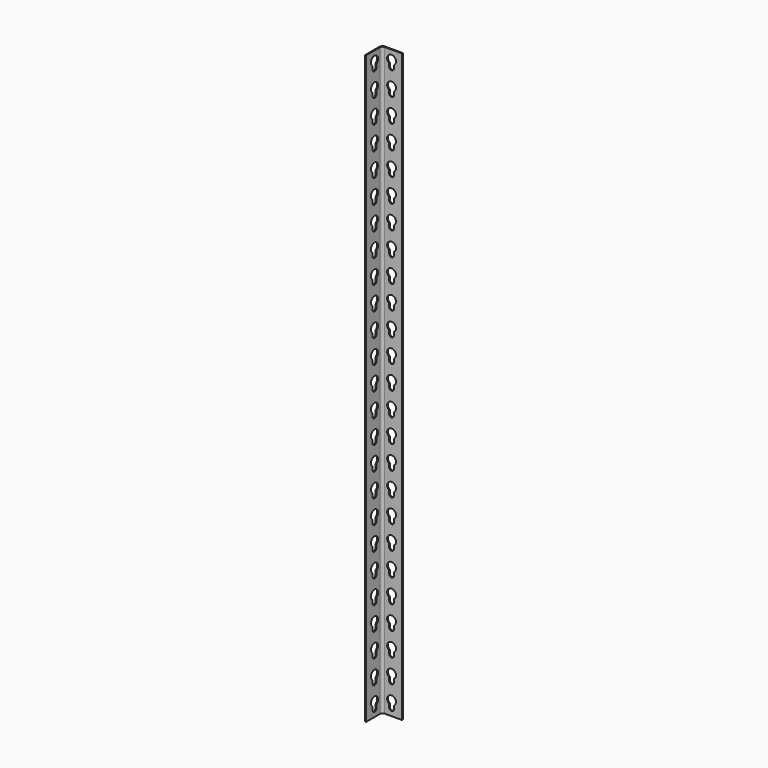
from build123d import *

# Parameters (mm, degrees)
F1_DEPTH = 914
F3_DEPTH = 1.5
F4_ANGLE = 90
F7_R     = 4
F8_R     = 5


with BuildPart() as f1:
    # F0 (on Top) → F1 (new body)
    with BuildSketch(Plane.XY):
        Polygon((-1.5, 1.5), (-1.5, 0), (0, 0), (31, 0), (31, 1.5), align=None)
    extrude(amount=F1_DEPTH)

    # F2 (on face) → F3 (cut, through all)
    with BuildSketch(Plane.XZ):
        with BuildLine():
            ThreePointArc((11.05, 10.8), (14.75, 7.1), (18.45, 10.8))
            Line((18.45, 10.8), (18.45, 15.8))
            ThreePointArc((18.45, 15.8), (14.75, 28.5119153836), (11.05, 15.8))
            Line((11.05, 15.8), (11.05, 10.8))
        make_face()
        with BuildLine():
            Line((11.05, 52.4), (11.05, 47.4))
            ThreePointArc((11.05, 47.4), (14.75, 43.7), (18.45, 47.4))
            Line((18.45, 47.4), (18.45, 52.4))
            ThreePointArc((18.45, 52.4), (14.75, 65.1119153836), (11.05, 52.4))
        make_face()
        with BuildLine():
            Line((11.05, 89), (11.05, 84))
            ThreePointArc((11.05, 84), (14.75, 80.3), (18.45, 84))
            Line((18.45, 84), (18.45, 89))
            ThreePointArc((18.45, 89), (14.75, 101.7119153836), (11.05, 89))
        make_face()
        with BuildLine():
            Line((11.05, 125.6), (11.05, 120.6))
            ThreePointArc((11.05, 120.6), (14.75, 116.9), (18.45, 120.6))
            Line((18.45, 120.6), (18.45, 125.6))
            ThreePointArc((18.45, 125.6), (14.75, 138.3119153836), (11.05, 125.6))
        make_face()
        with BuildLine():
            Line((11.05, 162.2), (11.05, 157.2))
            ThreePointArc((11.05, 157.2), (14.75, 153.5), (18.45, 157.2))
            Line((18.45, 157.2), (18.45, 162.2))
            ThreePointArc((18.45, 162.2), (14.75, 174.9119153836), (11.05, 162.2))
        make_face()
        with BuildLine():
            Line((11.05, 198.8), (11.05, 193.8))
            ThreePointArc((11.05, 193.8), (14.75, 190.1), (18.45, 193.8))
            Line((18.45, 193.8), (18.45, 198.8))
            ThreePointArc((18.45, 198.8), (14.75, 211.5119153836), (11.05, 198.8))
        make_face()
        with BuildLine():
            Line((11.05, 235.4), (11.05, 230.4))
            ThreePointArc((11.05, 230.4), (14.75, 226.7), (18.45, 230.4))
            Line((18.45, 230.4), (18.45, 235.4))
            ThreePointArc((18.45, 235.4), (14.75, 248.1119153836), (11.05, 235.4))
        make_face()
        with BuildLine():
            Line((11.05, 272), (11.05, 267))
            ThreePointArc((11.05, 267), (14.75, 263.3), (18.45, 267))
            Line((18.45, 267), (18.45, 272))
            ThreePointArc((18.45, 272), (14.75, 284.7119153836), (11.05, 272))
        make_face()
        with BuildLine():
            Line((11.05, 308.6), (11.05, 303.6))
            ThreePointArc((11.05, 303.6), (14.75, 299.9), (18.45, 303.6))
            Line((18.45, 303.6), (18.45, 308.6))
            ThreePointArc((18.45, 308.6), (14.75, 321.3119153836), (11.05, 308.6))
        make_face()
        with BuildLine():
            Line((11.05, 345.2), (11.05, 340.2))
            ThreePointArc((11.05, 340.2), (14.75, 336.5), (18.45, 340.2))
            Line((18.45, 340.2), (18.45, 345.2))
            ThreePointArc((18.45, 345.2), (14.75, 357.9119153836), (11.05, 345.2))
        make_face()
        with BuildLine():
            Line((11.05, 381.8), (11.05, 376.8))
            ThreePointArc((11.05, 376.8), (14.75, 373.1), (18.45, 376.8))
            Line((18.45, 376.8), (18.45, 381.8))
            ThreePointArc((18.45, 381.8), (14.75, 394.5119153836), (11.05, 381.8))
        make_face()
        with BuildLine():
            Line((11.05, 418.4), (11.05, 413.4))
            ThreePointArc((11.05, 413.4), (14.75, 409.7), (18.45, 413.4))
            Line((18.45, 413.4), (18.45, 418.4))
            ThreePointArc((18.45, 418.4), (14.75, 431.1119153836), (11.05, 418.4))
        make_face()
        with BuildLine():
            Line((11.05, 455), (11.05, 450))
            ThreePointArc((11.05, 450), (14.75, 446.3), (18.45, 450))
            Line((18.45, 450), (18.45, 455))
            ThreePointArc((18.45, 455), (14.75, 467.7119153836), (11.05, 455))
        make_face()
        with BuildLine():
            Line((11.05, 491.6), (11.05, 486.6))
            ThreePointArc((11.05, 486.6), (14.75, 482.9), (18.45, 486.6))
            Line((18.45, 486.6), (18.45, 491.6))
            ThreePointArc((18.45, 491.6), (14.75, 504.3119153836), (11.05, 491.6))
        make_face()
        with BuildLine():
            Line((11.05, 528.2), (11.05, 523.2))
            ThreePointArc((11.05, 523.2), (14.75, 519.5), (18.45, 523.2))
            Line((18.45, 523.2), (18.45, 528.2))
            ThreePointArc((18.45, 528.2), (14.75, 540.9119153836), (11.05, 528.2))
        make_face()
        with BuildLine():
            Line((11.05, 564.8), (11.05, 559.8))
            ThreePointArc((11.05, 559.8), (14.75, 556.1), (18.45, 559.8))
            Line((18.45, 559.8), (18.45, 564.8))
            ThreePointArc((18.45, 564.8), (14.75, 577.5119153836), (11.05, 564.8))
        make_face()
        with BuildLine():
            Line((11.05, 601.4), (11.05, 596.4))
            ThreePointArc((11.05, 596.4), (14.75, 592.7), (18.45, 596.4))
            Line((18.45, 596.4), (18.45, 601.4))
            ThreePointArc((18.45, 601.4), (14.75, 614.1119153836), (11.05, 601.4))
        make_face()
        with BuildLine():
            Line((11.05, 638), (11.05, 633))
            ThreePointArc((11.05, 633), (14.75, 629.3), (18.45, 633))
            Line((18.45, 633), (18.45, 638))
            ThreePointArc((18.45, 638), (14.75, 650.7119153836), (11.05, 638))
        make_face()
        with BuildLine():
            Line((11.05, 674.6), (11.05, 669.6))
            ThreePointArc((11.05, 669.6), (14.75, 665.9), (18.45, 669.6))
            Line((18.45, 669.6), (18.45, 674.6))
            ThreePointArc((18.45, 674.6), (14.75, 687.3119153836), (11.05, 674.6))
        make_face()
        with BuildLine():
            Line((11.05, 711.2), (11.05, 706.2))
            ThreePointArc((11.05, 706.2), (14.75, 702.5), (18.45, 706.2))
            Line((18.45, 706.2), (18.45, 711.2))
            ThreePointArc((18.45, 711.2), (14.75, 723.9119153836), (11.05, 711.2))
        make_face()
        with BuildLine():
            Line((11.05, 747.8), (11.05, 742.8))
            ThreePointArc((11.05, 742.8), (14.75, 739.1), (18.45, 742.8))
            Line((18.45, 742.8), (18.45, 747.8))
            ThreePointArc((18.45, 747.8), (14.75, 760.5119153836), (11.05, 747.8))
        make_face()
        with BuildLine():
            Line((11.05, 784.4), (11.05, 779.4))
            ThreePointArc((11.05, 779.4), (14.75, 775.7), (18.45, 779.4))
            Line((18.45, 779.4), (18.45, 784.4))
            ThreePointArc((18.45, 784.4), (14.75, 797.1119153836), (11.05, 784.4))
        make_face()
        with BuildLine():
            Line((11.05, 821), (11.05, 816))
            ThreePointArc((11.05, 816), (14.75, 812.3), (18.45, 816))
            Line((18.45, 816), (18.45, 821))
            ThreePointArc((18.45, 821), (14.75, 833.7119153836), (11.05, 821))
        make_face()
        with BuildLine():
            Line((11.05, 857.6), (11.05, 852.6))
            ThreePointArc((11.05, 852.6), (14.75, 848.9), (18.45, 852.6))
            Line((18.45, 852.6), (18.45, 857.6))
            ThreePointArc((18.45, 857.6), (14.75, 870.3119153836), (11.05, 857.6))
        make_face()
        with BuildLine():
            Line((11.05, 894.2), (11.05, 889.2))
            ThreePointArc((11.05, 889.2), (14.75, 885.5), (18.45, 889.2))
            Line((18.45, 889.2), (18.45, 894.2))
            ThreePointArc((18.45, 894.2), (14.75, 906.9119153836), (11.05, 894.2))
        make_face()
    extrude(amount=-F3_DEPTH, mode=Mode.SUBTRACT)


with BuildPart() as f4_1:
    # F4: copy of F1
    add(f1.part.rotate(Axis((-1.5, 0, 457), (0, 0, -1)), F4_ANGLE))


with BuildPart() as f4_1_1:
    # F5: moved
    add(f4_1.part.moved(Location((0, 1.5, 0))))

    # F6: union F1
    add(f1.part)

    # F7
    f7_edges = [f4_1_1.edges().sort_by_distance(p)[0] for p in [
        (0, 0, 457),
    ]]
    fillet(f7_edges, radius=F7_R)

    # F8
    f8_edges = [f4_1_1.edges().sort_by_distance(p)[0] for p in [
        (-1.5, 1.5, 457),
    ]]
    fillet(f8_edges, radius=F8_R)


solid = f4_1_1.part
